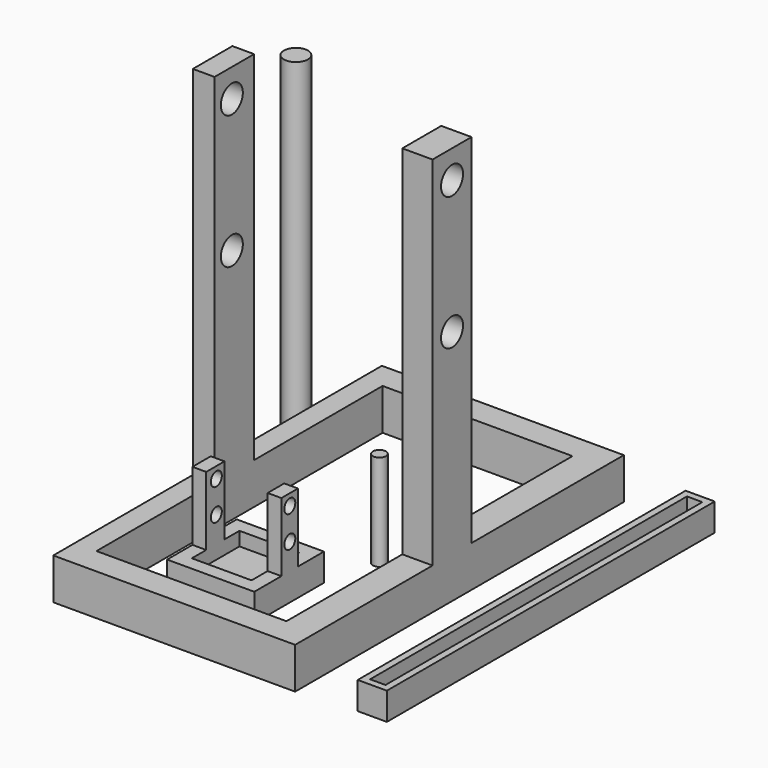
from build123d import *

# Parameters (mm, degrees)
F0_W      = 99.0480743349
F0_H      = 131.0261934996
F1_DEPTH  = 25
F3_D      = 80
F4_W      = 10.3947483003
F4_H      = 28.5077588633
F5_DEPTH  = 55
F7_D      = 10
F8_R      = 4.3865377981
F9_DEPTH  = 120
F10_DEPTH = 60
F12_D     = 10
F13_DEPTH = 5
F14_DEPTH = 5
F15_DEPTH = 5
F16_DEPTH = 10
F17_DEPTH = 10
F18_W     = 10.6056071818
F18_H     = 149.0600779653
F19_DEPTH = 10
F20_T     = -2.5
F20_2_T   = -2.5
F22_W     = 7.8981034458
F22_H     = 8.4575563669
F22_H_2   = 130.0605162978
F22_H_3   = 9.5668360591
F22_W_2   = 69.0817683935
F22_W_3   = 11.004479602
F22_H_4   = 9.7881406546
F23_DEPTH = 15
F24_W     = 7.8981034458
F24_H     = 17.9785350338
F24_W_2   = 11.004479602
F24_H_2   = 17.717437353
F25_DEPTH = 130
F27_D     = 10
F28_W     = 31.7221675068
F28_H     = 31.6584389657
F29_DEPTH = 5
F30_DEPTH = 5
F31_T     = -5
F32_W     = 5
F32_H     = 8.3243623376
F32_H_2   = 7.5445622206
F33_DEPTH = 25
F35_D     = 5
F36_R     = 2.375
F37_DEPTH = 35


# Not quite as in the source:
# - a shell that OpenCascade refuses in one call is made with other operations: the cavity is built on its own and cut out
# - a feature names something its author has since deleted; it is built from what else it names


with BuildPart() as f1:
    # F0 (on Top) → F1 (new body)
    with BuildSketch(Plane.XY):
        with Locations((-1.6936603934, -0.8678138256)):
            Rectangle(F0_W, F0_H)
    extrude(amount=F1_DEPTH)

    # F3 (through all)
    with Locations(Plane.XY.offset(25)):
        with Locations((0, 1.7684714403)):
            Hole(F3_D / 2)

    # F4 (on face) → F5 (join)
    with BuildSketch(Plane.XY.offset(25)):
        with Locations((-46.0203234106, -0.7940088399)):
            Rectangle(F4_W, F4_H)
        with BuildLine():
            Line((47.8303767741, -17.6419820637), (47.8303767741, 13.5616535332))
            Line((47.8303767741, 13.5616535332), (38.2219944027, 13.5616535332))
            ThreePointArc((38.2219944027, 13.5616535332), (39.5530009994, 7.7317014329), (40, 1.7684714403))
            ThreePointArc((40, 1.7684714403), (39.5530009994, -4.1947585523), (38.2219944027, -10.0247106526))
            Line((38.2219944027, -10.0247106526), (38.2219944027, -17.6419820637))
            Line((38.2219944027, -17.6419820637), (47.8303767741, -17.6419820637))
        make_face()
    extrude(amount=F5_DEPTH)

    # F7 (through all)
    with Locations(Plane(origin=(-51.2176975608, 0, 0), x_dir=(0, -1, 0), z_dir=(-1, 0, 0))):
        with Locations((0, 69.6488469839)):
            Hole(F7_D / 2)

    # F10 (add): a face of the model
    f10_faces = [f1.faces().sort_by_distance(p)[0] for p in [
        (-46.0203234106, -0.7940088399, 80),
    ]]
    extrude(f10_faces, amount=F10_DEPTH)

    # F12 (through all)
    with Locations(Plane(origin=(-51.2176975608, 0, 0), x_dir=(0, -1, 0), z_dir=(-1, 0, 0))):
        with Locations((0, 129.8670172691)):
            Hole(F12_D / 2)

    # F13 (add): a face of the model
    f13_faces = [f1.faces().sort_by_distance(p)[0] for p in [
        (-46.0203234106, -15.0478882715, 82.5),
    ]]
    extrude(f13_faces, amount=-F13_DEPTH)

    # F14 (add): a face of the model
    f14_faces = [f1.faces().sort_by_distance(p)[0] for p in [
        (43.0261855884, -17.6419820637, 52.5),
    ]]
    extrude(f14_faces, amount=-F14_DEPTH)

    # F15 (add): a face of the model
    f15_faces = [f1.faces().sort_by_distance(p)[0] for p in [
        (46.1878669746, 39.1034682287, 25),
    ]]
    extrude(f15_faces, amount=-F15_DEPTH)

    # F16 (add): a face of the model
    f16_faces = [f1.faces().sort_by_distance(p)[0] for p in [
        (46.1878669746, 39.1034682287, 25),
    ]]
    extrude(f16_faces, amount=-F16_DEPTH)

    # F17 (add): a face of the model
    f17_faces = [f1.faces().sort_by_distance(p)[0] for p in [
        (46.1878669746, 39.1034682287, 25),
    ]]
    extrude(f17_faces, amount=-F17_DEPTH)

    # F20#2: a shell. OpenCascade refuses it in one call, so the cavity is built on its own and cut out:
    # the body offset inwards by the wall thickness, plus a prism from it out through each open face.
    f20_2_core = offset(f1.part, amount=F20_2_T, mode=Mode.PRIVATE)
    f20_2_exits = [f20_2_core.faces().sort_by_distance(p)[0] for p in [
        (-2.773323, -45.938788, 22.5),
        (-2.856032, 45.670287, 22.5),
    ]]
    add(f20_2_core, mode=Mode.SUBTRACT)
    extrude(f20_2_exits, amount=-F20_2_T, mode=Mode.SUBTRACT)


with BuildPart() as f9:
    # F8 (on Top) → F9 (new body)
    with BuildSketch(Plane.XY):
        with Locations((-69.7542577982, 49.2088384926)):
            Circle(F8_R)
    extrude(amount=F9_DEPTH)


with BuildPart() as f19:
    # F18 (on Top) → F19 (new body)
    with BuildSketch(Plane.XY):
        with Locations((57.3895256966, -0.4549883306)):
            Rectangle(F18_W, F18_H)
    extrude(amount=F19_DEPTH)

    # F20
    f20_openings = [f19.faces().sort_by_distance(p)[0] for p in [
        (57.389526, -0.454988, 10),
    ]]
    offset(amount=F20_T, openings=f20_openings)


with BuildPart() as f23:
    # F22 (on Top) → F23 (new body)
    with BuildSketch(Plane.XY):
        Polygon((-49.3639744818, -75.395129621), (-57.2620779276, -75.395129621), (-57.2620779276, -76.7257139087), (19.7177939117, -76.7257139087), (19.7177939117, -66.9375732541), (-49.3639744818, -66.9375732541), align=None)
        with Locations((-53.3130262047, -71.1663514376)):
            Rectangle(F22_W, F22_H)
        with Locations((-53.3130262047, -1.9073151052)):
            Rectangle(F22_W, F22_H_2)
        with Locations((-53.3130262047, 67.9063610733)):
            Rectangle(F22_W, F22_H_3)
        with Locations((-14.8230902851, 67.9063610733)):
            Rectangle(F22_W_2, F22_H_3)
        with Locations((25.2200337127, 67.9063610733)):
            Rectangle(F22_W_3, F22_H_3)
        with Locations((25.2200337127, -1.9073151052)):
            Rectangle(F22_W_3, F22_H_2)
        with Locations((25.2200337127, -71.8316435814)):
            Rectangle(F22_W_3, F22_H_4)
    extrude(amount=F23_DEPTH)

    # F24 (on face) → F25 (join)
    with BuildSketch(Plane.XY.offset(15)):
        with Locations((-53.3130262047, -4.2759669013)):
            Rectangle(F24_W, F24_H)
        with Locations((25.2200337127, -5.4010595195)):
            Rectangle(F24_W_2, F24_H_2)
    extrude(amount=F25_DEPTH)

    # F27 (through all)
    with Locations(Plane.YZ.offset(30.7222735137)):
        with Locations((-5.4010595195, 134.7581446171), (-5.4010595195, 86.2278193235)):
            Hole(F27_D / 2)


with BuildPart() as f29:
    # F28 (on Top) → F29 (new body)
    with BuildSketch(Plane.XY):
        with Locations((-20.5884641036, -35.1668419316)):
            Rectangle(F28_W, F28_H)
    extrude(amount=F29_DEPTH)

    # F30 (add): a face of the model
    f30_faces = [f29.faces().sort_by_distance(p)[0] for p in [
        (-20.5884641036, -35.1668419316, 5),
    ]]
    extrude(f30_faces, amount=F30_DEPTH)

    # F31
    f31_openings = [f29.faces().sort_by_distance(p)[0] for p in [
        (-20.588464, -35.166842, 10),
    ]]
    offset(amount=F31_T, openings=f31_openings)

    # F32 (on face) → F33 (join)
    with BuildSketch(Plane.XY.offset(10)):
        with Locations((-33.949547857, -35.2967381477)):
            Rectangle(F32_W, F32_H)
        with Locations((-7.2273803502, -34.9068380892)):
            Rectangle(F32_W, F32_H_2)
    extrude(amount=F33_DEPTH)

    # F35 (through all)
    with Locations(Plane.YZ.offset(-4.7273803502)):
        with Locations((-34.8523966968, 30.9046246111), (-34.8523966968, 19.4699745625)):
            Hole(F35_D / 2)


with BuildPart() as f37:
    # F36 (on Top) → F37 (new body)
    with BuildSketch(Plane.XY):
        Circle(F36_R)
    extrude(amount=F37_DEPTH)


solid = Compound([f9.part, f19.part, f23.part, f29.part, f37.part])
